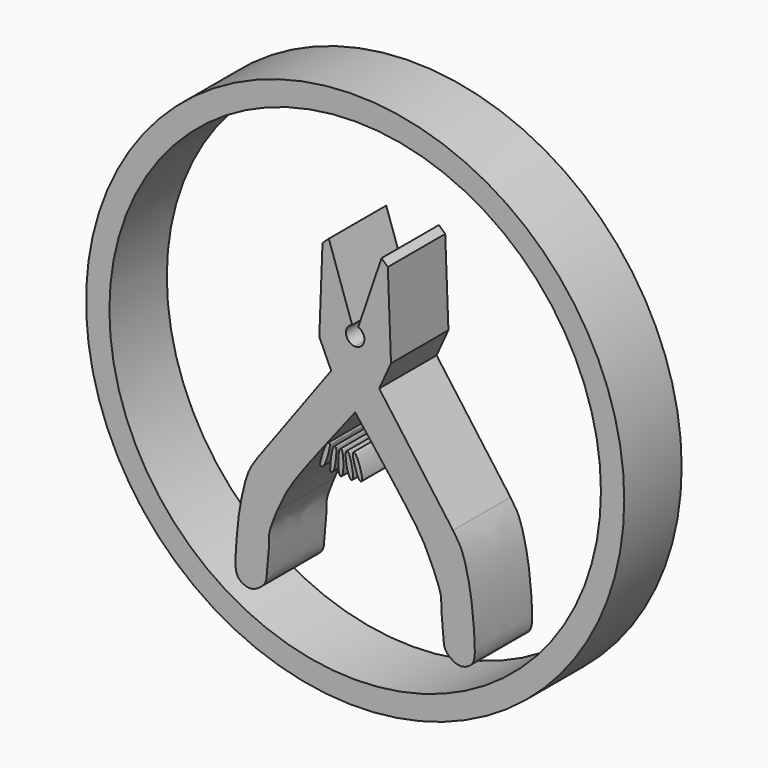
from build123d import *

# Parameters (mm, degrees)
F0_R     = 75
F0_R_2   = 68.5
F3_DEPTH = 20
F4_DEPTH = 20
F5_DEPTH = 25


# Not quite as in the source:
# - the program builds the solid bodies; features that only make, move or delete a surface that nothing else refers to are left out


with BuildPart() as f3:
    # F0 (on Front) → F3 (new body)
    with BuildSketch(Plane.XZ):
        Circle(F0_R)
        Circle(F0_R_2, mode=Mode.SUBTRACT)
    extrude(amount=F3_DEPTH)


with BuildPart() as f4:
    # F1 (on Front) → F4 (new body)
    with BuildSketch(Plane.XZ):
        with BuildLine():
            Line((-9.0995086357, 35.7137694955), (-9.9920583889, 12.3855927959))
            Line((-9.9920583889, 12.3855927959), (-6.6928253509, 5.1298425533))
            Line((-6.6928253509, 5.1298425533), (-27.2733609587, -22.9763794423))
            add(Edge.make_bspline(
                [(-27.2733609587, -22.9763794423), (-28.0701572192, -24.1113172157), (-29.7872293545, -26.5540850688), (-31.2685830075, -32.0626437011), (-32.2245036764, -36.8943208623), (-32.9847834531, -42.7925387191), (-33.158807326, -46.8342729752), (-33.6305868752, -52.7804458081), (-31.9328109038, -54.9564916282), (-29.1769791488, -55.9719408417), (-26.6229388074, -54.7266613513), (-24.7400791093, -52.7872522334), (-24.6867835743, -50.4482589336), (-23.8091970418, -43.7699607903), (-24.295828176, -39.8589629216), (-22.549959608, -36.3023901443), (-21.8346624254, -34.3259416133)],
                knots=[0, 0, 0, 0, 0.072807798, 0.1555955303, 0.2349482052, 0.3188790992, 0.3920771862, 0.4755345455, 0.5311831014, 0.5880551952, 0.6460190998, 0.7009696888, 0.7541334009, 0.8440572518, 0.9149232468, 1, 1, 1, 1], degree=3))
            add(Edge.make_bspline(
                [(-21.8346624254, -34.3259416133), (-21.1977907958, -33.16729403), (-20.1480574173, -30.456005728), (-17.1283124622, -24.7557830955), (-6.9783833146, -11.8166051914), (0, -2.868756419)],
                knots=[0, 0, 0, 0, 0.2032576565, 0.4518618851, 1, 1, 1, 1], degree=3))
            Line((0, -2.868756419), (0, 13.2500697194))
            ThreePointArc((0, 13.2500697194), (-2.5411327705, 15.3983203428), (-0.8456606301, 18.2614848018))
            Line((-0.8456606301, 18.2614848018), (-7.3425769806, 37.3269505799))
            Line((-7.3425769806, 37.3269505799), (-9.0995086357, 35.7137694955))
        make_face()
        with BuildLine():
            ThreePointArc((0.8456606301, 18.2614848018), (2.5411327705, 15.3983203428), (0, 13.2500697194))
            Line((0, 13.2500697194), (0, -2.868756419))
            add(Edge.make_bspline(
                [(21.8346624254, -34.3259416133), (21.1977907958, -33.16729403), (20.1480574173, -30.456005728), (17.1283124622, -24.7557830955), (6.9783833146, -11.8166051914), (0, -2.868756419)],
                knots=[0, 0, 0, 0, 0.2032576565, 0.4518618851, 1, 1, 1, 1], degree=3))
            add(Edge.make_bspline(
                [(27.2733609587, -22.9763794423), (28.0701572192, -24.1113172157), (29.7872293545, -26.5540850688), (31.2685830075, -32.0626437011), (32.2245036764, -36.8943208623), (32.9847834531, -42.7925387191), (33.158807326, -46.8342729752), (33.6305868752, -52.7804458081), (31.9328109038, -54.9564916282), (29.1769791488, -55.9719408417), (26.6229388074, -54.7266613513), (24.7400791093, -52.7872522334), (24.6867835743, -50.4482589336), (23.8091970418, -43.7699607903), (24.295828176, -39.8589629216), (22.549959608, -36.3023901443), (21.8346624254, -34.3259416133)],
                knots=[0, 0, 0, 0, 0.072807798, 0.1555955303, 0.2349482052, 0.3188790992, 0.3920771862, 0.4755345455, 0.5311831014, 0.5880551952, 0.6460190998, 0.7009696888, 0.7541334009, 0.8440572518, 0.9149232468, 1, 1, 1, 1], degree=3))
            Line((27.2733609587, -22.9763794423), (6.6928253509, 5.1298425533))
            Line((6.6928253509, 5.1298425533), (9.9920583889, 12.3855927959))
            Line((9.9920583889, 12.3855927959), (9.0995086357, 35.7137694955))
            Line((9.0995086357, 35.7137694955), (7.3425769806, 37.3269505799))
            Line((7.3425769806, 37.3269505799), (0.8456606301, 18.2614848018))
        make_face()
    extrude(amount=F4_DEPTH)


with BuildPart() as f5:
    # F2 (on Front) → F5 (new body)
    with BuildSketch(Plane.XZ):
        with BuildLine():
            add(Edge.make_bspline(
                [(-3.979253338, -9.9576336976), (-4.7234029968, -11.020130225), (-5.8184468002, -14.9108947774), (-5.7897516039, -15.9524187409), (-4.3693884753, -15.7940391734), (-2.8935100281, -10.3328801035), (-3.0911885315, -9.2502342639), (-3.6684479768, -9.5138659513), (-3.979253338, -9.9576336976)],
                knots=[0, 0, 0, 0, 0.2780047915, 0.3842955615, 0.4939509538, 0.7783698483, 0.8838870936, 1, 1, 1, 1], degree=3))
        make_face()
    extrude(amount=F5_DEPTH)


with BuildPart() as f5b:
    # F2 (on Front) → F5, piece 2 (new body)
    with BuildSketch(Plane.XZ):
        with BuildLine():
            add(Edge.make_bspline(
                [(-2.1406578188, -10.2233118998), (-2.6474458062, -11.3166308025), (-3.0338956059, -15.4694728402), (-2.9289606035, -16.5348183601), (-1.5817817155, -16.0908600995), (-1.0340360871, -10.4368448604), (-1.5052646067, -9.5319348747), (-1.9480069005, -9.8076965028), (-2.1406578188, -10.2233118998)],
                knots=[0, 0, 0, 0, 0.2824524627, 0.3913703426, 0.5013182062, 0.7892651608, 0.8926282239, 1, 1, 1, 1], degree=3))
        make_face()
    extrude(amount=F5_DEPTH)


with BuildPart() as f5c:
    # F2 (on Front) → F5, piece 3 (new body)
    with BuildSketch(Plane.XZ):
        with BuildLine():
            add(Edge.make_bspline(
                [(-0.4428708344, -10.4359230027), (-0.7679443068, -11.6027928695), (-0.8129996926, -15.8735305643), (-0.0092816936, -16.7627087867), (0.8490072939, -15.937818454), (0.759733332, -10.4292701958), (-0.0030141921, -9.6638237199), (-0.3223258254, -10.0032197818), (-0.4428708344, -10.4359230027)],
                knots=[0, 0, 0, 0, 0.2843492762, 0.3954718988, 0.5043563334, 0.7906022123, 0.8945564958, 1, 1, 1, 1], degree=3))
        make_face()
    extrude(amount=F5_DEPTH)


with BuildPart() as f5d:
    # F2 (on Front) → F5, piece 4 (new body)
    with BuildSketch(Plane.XZ):
        with BuildLine():
            add(Edge.make_bspline(
                [(1.3673621106, -10.6255200318), (1.2564075628, -11.9354456348), (2.0140270441, -15.9035244545), (3.0804786381, -16.7230068951), (3.7254514579, -15.6336444386), (2.558694432, -10.3843869657), (1.7256497602, -9.521754608), (1.4142592239, -10.0718543126), (1.3673621106, -10.6255200318)],
                knots=[0, 0, 0, 0, 0.2749070885, 0.3890790555, 0.4983250276, 0.7771368273, 0.8838051332, 1, 1, 1, 1], degree=3))
        make_face()
    extrude(amount=F5_DEPTH)


with BuildPart() as f5e:
    # F2 (on Front) → F5, piece 5 (new body)
    with BuildSketch(Plane.XZ):
        with BuildLine():
            add(Edge.make_bspline(
                [(3.3727246337, -10.2085033432), (3.4403839991, -11.4169141621), (4.5571836092, -15.3596231402), (5.6356497321, -16.2493912459), (6.2925703598, -15.1500632705), (4.5332733528, -9.8337640221), (3.5031655273, -9.2729109296), (3.3467951481, -9.7453971539), (3.3727246337, -10.2085033432)],
                knots=[0, 0, 0, 0, 0.2765236536, 0.3967819627, 0.5046019431, 0.7887525835, 0.8940262587, 1, 1, 1, 1], degree=3))
        make_face()
    extrude(amount=F5_DEPTH)


solid = Compound([f3.part, f4.part, f5.part, f5b.part, f5c.part, f5d.part, f5e.part])
